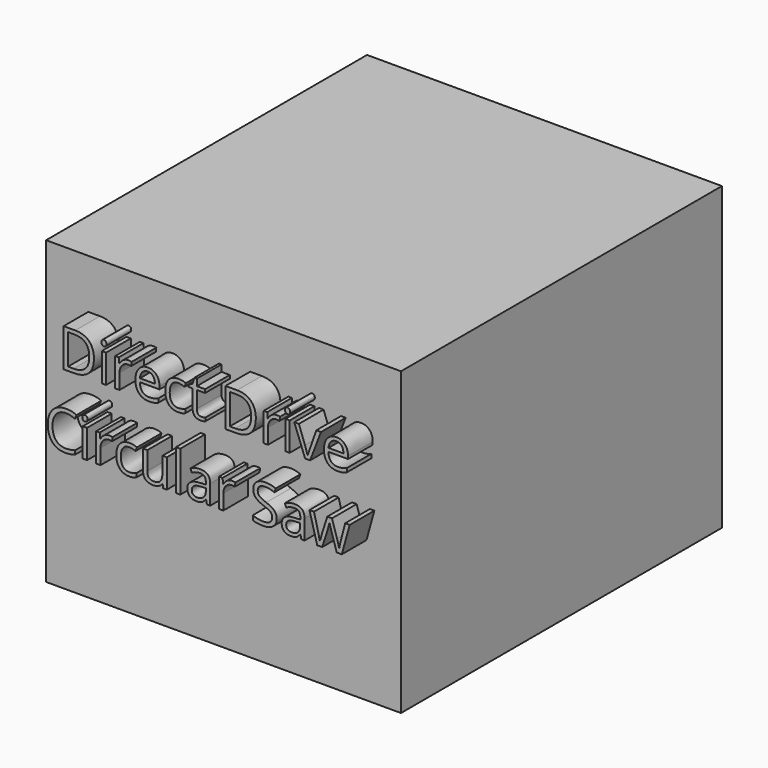
from build123d import *

# Parameters (mm, degrees)
F0_W         = 292.1
F0_H         = 247.65
F1_DEPTH     = 330.2
F2_TEXT_SIZE = 43.8226176035
F3_DEPTH     = 25.4


# Not quite as in the source:
# - Text() gives the source's letters only with a copy of the font that has no kerning and outlines rounded to 1/6400 em; it was checked with that copy


with BuildPart() as f1:
    # F0 (on Front) → F1 (new body)
    with BuildSketch(Plane.XZ):
        Rectangle(F0_W, F0_H)
    extrude(amount=F1_DEPTH)

    # F2 (on face) → F3 (join)
    with BuildSketch(Plane.XZ.offset(330.2)):
        with Locations((-115.6129667071, 51.8868514291)):
            Text('Direct Drive', F2_TEXT_SIZE, font='Open Sans', text_align=(TextAlign.LEFT, TextAlign.BOTTOM))
        with Locations((-127, -7.7119085116)):
            Text('Circular Saw', F2_TEXT_SIZE, font='Open Sans', text_align=(TextAlign.LEFT, TextAlign.BOTTOM))
    extrude(amount=F3_DEPTH)


solid = f1.part
